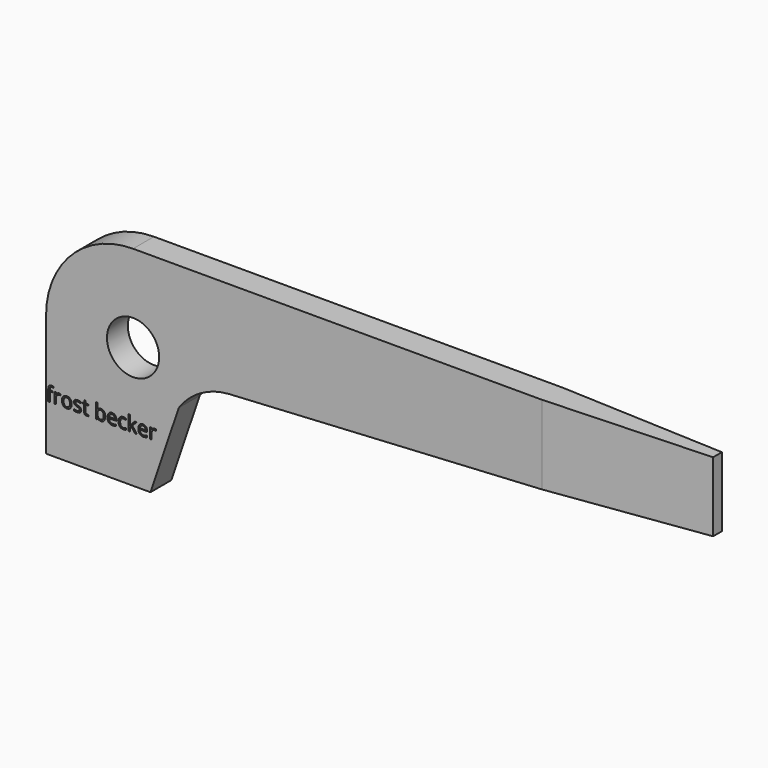
from build123d import *

# Parameters (mm, degrees)
F1_DEPTH     = 2.38125
F2_R         = 2.38125
F3_DEPTH     = 2.38225
F5_DEPTH     = 25.4
F6_TEXT_SIZE = 1.8013182169
F7_DEPTH     = 2.54


# Not quite as in the source:
# - a feature names something its author has since deleted; it is built from what else it names
# - Text() gives the source's letters only with a copy of the font that has no kerning and outlines rounded to 1/6400 em; it was checked with that copy


with BuildPart() as f1:
    # F0 (on Front) → F1 (new body)
    with BuildSketch(Plane.XZ):
        with BuildLine():
            Line((60.325, 19.05), (7.9375, 19.05))
            ThreePointArc((7.9375, 19.05), (2.3248399243, 16.7251600757), (0, 11.1125))
            Line((0, 11.1125), (0, 0))
            Line((0, 0), (9.525, 0))
            Line((9.525, 0), (12.1103451907, 7.6262422093))
            ThreePointArc((12.1103451907, 7.6262422093), (14.1301474138, 9.462992063), (16.7510204416, 10.2273712997))
            Line((16.7510204416, 10.2273712997), (60.325, 12.7))
            Line((60.325, 12.7), (60.325, 19.05))
        make_face()
    extrude(amount=F1_DEPTH)

    # F2 (on face) → F3 (cut, through all)
    with BuildSketch(Plane.XZ.offset(2.38125)):
        with Locations((7.9375, 11.1125)):
            Circle(F2_R)
    extrude(amount=-F3_DEPTH, mode=Mode.SUBTRACT)

    # F4 (on face) → F5 (cut)
    with BuildSketch(Plane.XY.offset(19.05)):
        Polygon((60.325, -2.38125), (60.325, -1.6947635135), (45.24375, -2.38125), align=None)
        Polygon((60.325, 0), (45.24375, 0), (60.325, -0.6864864865), align=None)
    extrude(amount=-F5_DEPTH, mode=Mode.SUBTRACT)

    # F6 (on face) → F7 (cut)
    with BuildSketch(Plane.XZ.offset(2.38125)):
        with Locations((0, 4.2593008839)):
            Text('frost becker', F6_TEXT_SIZE, font='Open Sans', text_align=(TextAlign.LEFT, TextAlign.BOTTOM))
    extrude(amount=-F7_DEPTH, mode=Mode.SUBTRACT)


solid = f1.part
